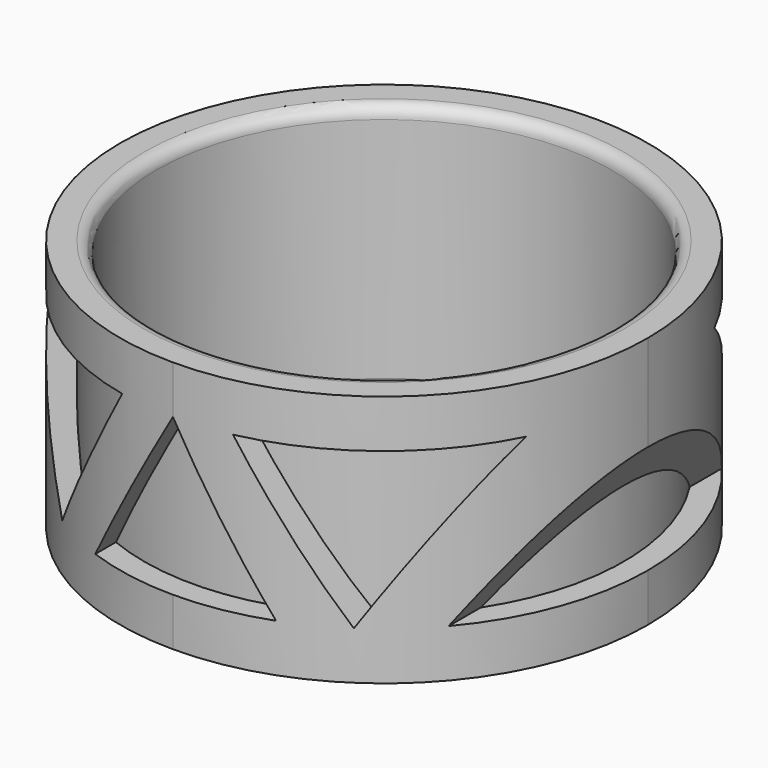
from build123d import *
from build123d import SkipClean  # not in build123d's __all__

# Parameters (mm, degrees)
F1_DEPTH = 22
F2_R     = 10
F2_R_2   = 9.5
F3_DEPTH = 25
F4_DEPTH = 10.5
F5_R     = 0.49999


# Not quite as in the source:
# - a fillet or chamfer is up to 0.001 mm smaller than in the source, because OpenCascade refuses the exact size


with BuildPart() as f1:
    # F0 (on Front) → F1 (new body)
    with BuildSketch(Plane.XZ):
        Polygon((-0.1671048567, 13.8939016994), (2.4461437974, 9.3676222578), (4.7555448741, 9.3676222578), (0.9875956817, 15.8939016994), (-0.1671048567, 15.8939016994), align=None)
        Polygon((0.9875956817, 15.8939016994), (8.5234940666, 15.8939016994), (9.678194605, 17.8939016994), (-0.1671048567, 17.8939016994), align=None)
        Polygon((9.678194605, 17.8939016994), (8.5234940666, 15.8939016994), (10.8328951433, 15.8939016994), align=None)
        Polygon((9.678194605, 17.8939016994), (10.8328951433, 15.8939016994), (11.9875956817, 17.8939016994), align=None)
        Polygon((11.9875956817, 17.8939016994), (10.8328951433, 15.8939016994), (13.1422962201, 15.8939016994), align=None)
        Polygon((-0.1671048567, 15.8939016994), (0.9875956817, 15.8939016994), (-0.1671048567, 17.8939016994), align=None)
        Polygon((13.1422962201, 15.8939016994), (20.678194605, 15.8939016994), (21.8328951433, 17.8939016994), (11.9875956817, 17.8939016994), align=None)
        Polygon((21.8328951433, 17.8939016994), (20.678194605, 15.8939016994), (21.8328951433, 15.8939016994), align=None)
        Polygon((20.678194605, 15.8939016994), (16.9102454125, 9.3676222578), (19.2196464893, 9.3676222578), (21.8328951433, 13.8939016994), (21.8328951433, 15.8939016994), align=None)
        Polygon((10.8328951433, 15.8939016994), (14.6008443358, 9.3676222578), (16.9102454125, 9.3676222578), (13.1422962201, 15.8939016994), align=None)
        Polygon((8.5234940666, 15.8939016994), (4.7555448741, 9.3676222578), (7.0649459509, 9.3676222578), (10.8328951433, 15.8939016994), align=None)
        Polygon((4.7555448741, 9.3676222578), (3.6008443358, 7.3676222578), (5.9102454125, 7.3676222578), align=None)
        Polygon((2.4461437974, 9.3676222578), (3.6008443358, 7.3676222578), (4.7555448741, 9.3676222578), align=None)
        Polygon((-0.1671048567, 9.3676222578), (-0.1671048567, 7.3676222578), (3.6008443358, 7.3676222578), (2.4461437974, 9.3676222578), align=None)
        Polygon((4.7555448741, 9.3676222578), (5.9102454125, 7.3676222578), (7.0649459509, 9.3676222578), align=None)
        Polygon((7.0649459509, 9.3676222578), (5.9102454125, 7.3676222578), (15.7555448741, 7.3676222578), (14.6008443358, 9.3676222578), align=None)
        Polygon((14.6008443358, 9.3676222578), (15.7555448741, 7.3676222578), (16.9102454125, 9.3676222578), align=None)
        Polygon((16.9102454125, 9.3676222578), (15.7555448741, 7.3676222578), (18.0649459509, 7.3676222578), align=None)
        Polygon((16.9102454125, 9.3676222578), (18.0649459509, 7.3676222578), (19.2196464893, 9.3676222578), align=None)
        Polygon((19.2196464893, 9.3676222578), (18.0649459509, 7.3676222578), (21.8328951433, 7.3676222578), (21.8328951433, 9.3676222578), align=None)
    extrude(amount=F1_DEPTH)

    # F2 (on face) → F3 (cut)
    with BuildSketch(Plane.XY.offset(17.8939016994)):
        with Locations((10.8328951433, -11)):
            Circle(F2_R)
        with Locations((10.8328951433, -11)):
            Circle(F2_R_2, mode=Mode.SUBTRACT)
        with Locations((10.8328951433, -11)):
            Circle(F2_R_2)
        with BuildLine():
            ThreePointArc((-0.1671048567, -11), (3.0547205503, -3.2218254069), (10.8328951433, 0))
            Line((10.8328951433, 0), (-0.1671048567, 0))
            Line((-0.1671048567, 0), (-0.1671048567, -11))
        make_face()
        with BuildLine():
            ThreePointArc((10.8328951433, 0), (18.6110697364, -3.2218254069), (21.8328951433, -11))
            Line((21.8328951433, -11), (21.8328951433, 0))
            Line((21.8328951433, 0), (10.8328951433, 0))
        make_face()
        with BuildLine():
            Line((21.8328951433, -22), (21.8328951433, -11))
            ThreePointArc((21.8328951433, -11), (18.6110697364, -18.7781745931), (10.8328951433, -22))
            Line((10.8328951433, -22), (21.8328951433, -22))
        make_face()
        with BuildLine():
            Line((-0.1671048567, -22), (10.8328951433, -22))
            ThreePointArc((10.8328951433, -22), (3.0547205503, -18.7781745931), (-0.1671048567, -11))
            Line((-0.1671048567, -11), (-0.1671048567, -22))
        make_face()
    with SkipClean():  # cleaning this boolean's faces spoils the solid; the shape is the same uncleaned
        extrude(amount=-F3_DEPTH, mode=Mode.SUBTRACT)

    # F2 (on face) → F4 (join)
    with BuildSketch(Plane.XY.offset(17.8939016994)):
        with Locations((10.8328951433, -11)):
            Circle(F2_R)
        with Locations((10.8328951433, -11)):
            Circle(F2_R_2, mode=Mode.SUBTRACT)
    with SkipClean():  # cleaning this boolean's faces spoils the solid; the shape is the same uncleaned
        extrude(amount=-F4_DEPTH)

    # F5 (radius 0.5 in the source; OpenCascade refuses exactly that, so slightly less here)
    f5_edges = [f1.edges().sort_by_distance(p)[0] for p in [
        (1.332895, -11, 7.393902),
        (1.332895, -11, 17.893902),
    ]]
    fillet(f5_edges, radius=F5_R)


solid = f1.part
